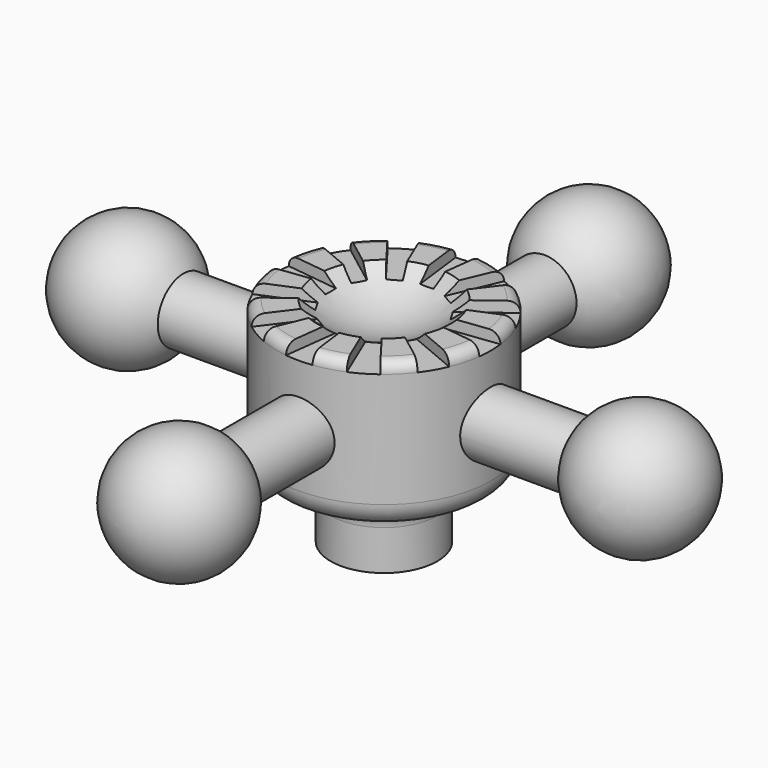
from build123d import *

# Parameters (mm, degrees)
F0_R            = 10
F1_DEPTH        = 7
F2_R            = 5
F3_DEPTH        = 6
F4_R            = 2.95
F5_DEPTH        = 9
F7_COPIES_COUNT = 4
F9_DEPTH        = 1
F9_COPIES_COUNT = 12
F12_R           = 2.25


# Not quite as in the source:
# - a pattern or mirror of a feature is missing from the dataset's text; its kind, count and spacing are read off the source's solid


with BuildPart() as f1:
    # F0 (on Top) → F1 (new body, symmetric)
    with BuildSketch(Plane.XY):
        Circle(F0_R)
    extrude(amount=F1_DEPTH, both=True)

    # F2 (on face) → F3 (join)
    with BuildSketch(Plane(origin=(0, 0, -7), x_dir=(1, 0, 0), z_dir=(0, 0, -1))):
        Circle(F2_R)
    extrude(amount=F3_DEPTH)

    # F4 (on face) → F5 (cut)
    with BuildSketch(Plane(origin=(0, 0, -13), x_dir=(1, 0, 0), z_dir=(0, 0, -1))):
        Circle(F4_R)
    extrude(amount=-F5_DEPTH, mode=Mode.SUBTRACT)

    # F6 (on Top) → F7 (revolve)
    with BuildSketch(Plane.XY):
        with BuildLine():
            Line((0, -30), (0, -9.5393920142))
            Line((0, -9.5393920142), (-3, -9.5393920142))
            Line((-3, -9.5393920142), (-3, -18.8038475773))
            ThreePointArc((-3, -18.8038475773), (-5.7955549577, -25.5529142706), (0, -30))
        make_face()
    f7 = revolve(axis=Axis((0, -23.260904476, 0), (0, -1, 0)))

    # F7_copies: F7 ×4 about axis
    f7_copies_axis = Axis((0, 0, 0), (0, 0, 1))
    for i in range(1, F7_COPIES_COUNT):
        add(f7.rotate(f7_copies_axis, i * 360 / F7_COPIES_COUNT))

    # F8 (on face) → F9 (cut)
    with BuildSketch(Plane.XY.offset(7)):
        Polygon((-0.625, -5), (-1.25, -10), (1.25, -10), (0.625, -5), align=None)
    f9 = extrude(amount=-F9_DEPTH, mode=Mode.SUBTRACT)

    # F9_copies: F9 ×12 about axis
    f9_copies_axis = Axis((0, 0, 0), (0, 0, 1))
    for i in range(1, F9_COPIES_COUNT):
        add(f9.rotate(f9_copies_axis, i * 360 / F9_COPIES_COUNT), mode=Mode.SUBTRACT)

    # F10 (on Front) → F11 (revolve, cut)
    with BuildSketch(Plane.XZ):
        with BuildLine():
            Line((0, 13.5833333333), (0, 4.5))
            ThreePointArc((0, 4.5), (3.6912057651, 5.283818622), (6.7453687816, 7.5))
            Line((6.7453687816, 7.5), (9, 7.5))
            Line((9, 7.5), (9, 7))
            ThreePointArc((9, 7), (9.7071067812, 6.7071067812), (10, 6))
            Line((10, 6), (12.8776788814, 6))
            Line((12.8776788814, 6), (0, 13.5833333333))
        make_face()
    revolve(axis=Axis((0, 0, 9.0416666667), (0, 0, 1)), mode=Mode.SUBTRACT)

    # F12
    f12_edges = [f1.edges().sort_by_distance(p)[0] for p in [
        (-10, 0, -7),
        (-5, 0, -7),
    ]]
    fillet(f12_edges, radius=F12_R)


solid = f1.part
